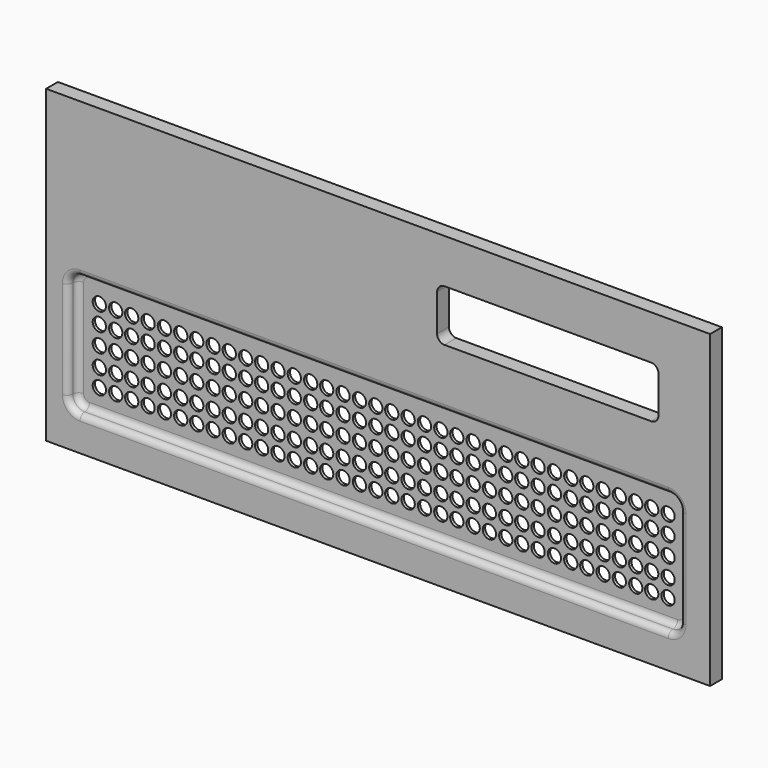
from build123d import *

# Parameters (mm, degrees)
F1_DEPTH = 10
F3_D     = 9
F4_D     = 9
F6_DEPTH = 8
F7_R     = 3.99999


# Not quite as in the source:
# - a fillet or chamfer is up to 0.001 mm smaller than in the source, because OpenCascade refuses the exact size
# - a feature names something its author has since deleted; it is built from what else it names


with BuildPart() as f1:
    # F0 (on Front) → F1 (new body)
    with BuildSketch(Plane.XZ):
        Polygon((0, 210), (0, 0), (450, 0), (450, 210), (265, 210), align=None)
        with BuildLine():
            Line((410, 145), (270, 145))
            ThreePointArc((270, 145), (266.4644660941, 146.4644660941), (265, 150))
            Line((265, 150), (265, 175))
            ThreePointArc((265, 175), (266.4644660941, 178.5355339059), (270, 180))
            Line((270, 180), (410, 180))
            ThreePointArc((410, 180), (413.5355339059, 178.5355339059), (415, 175))
            Line((415, 175), (415, 150))
            ThreePointArc((415, 150), (413.5355339059, 146.4644660941), (410, 145))
        make_face(mode=Mode.SUBTRACT)
    extrude(amount=F1_DEPTH)

    # F3 (through all)
    with Locations(Plane.XZ.offset(10)):
        with Locations((117.7525687963, 75.7827050984), (128.8482453674, 88.015531376), (73.7632680684, 38.015531376), (172.9213949293, 50.0800460577), (51.6047235578, 38.015531376), (150.7628504187, 38.015531376), (150.7628504187, 88.015531376), (128.8482453674, 75.7827050984), (117.7525687963, 38.015531376), (84.8589446396, 38.015531376), (84.8589446396, 63.015531376), (161.8257183582, 38.015531376), (95.6778731197, 75.7827050984), (172.9213949293, 63.015531376), (73.7632680684, 50.0800460577), (172.9213949293, 75.7827050984), (117.7525687963, 88.015531376), (128.8482453674, 38.015531376), (172.9213949293, 38.015531376), (161.8257183582, 63.015531376), (106.7735496908, 50.0800460577), (106.7735496908, 88.015531376), (40.7857950777, 63.015531376), (62.700400129, 63.015531376), (139.6671738476, 88.015531376), (117.7525687963, 50.0800460577), (139.6671738476, 63.015531376), (95.6778731197, 63.015531376), (161.8257183582, 75.7827050984), (106.7735496908, 38.015531376), (73.7632680684, 75.7827050984), (51.6047235578, 63.015531376), (172.9213949293, 88.015531376), (161.8257183582, 88.015531376), (84.8589446396, 75.7827050984), (128.8482453674, 63.015531376), (95.6778731197, 38.015531376), (84.8589446396, 88.015531376), (128.8482453674, 50.0800460577), (51.6047235578, 88.015531376), (62.700400129, 50.0800460577), (62.700400129, 75.7827050984), (51.6047235578, 75.7827050984), (106.7735496908, 63.015531376), (40.7857950777, 75.7827050984), (40.7857950777, 88.015531376), (40.7857950777, 50.0800460577), (29.6901185066, 50.0800460577), (29.6901185066, 63.015531376), (29.6901185066, 75.7827050984), (29.6901185066, 88.015531376), (29.6901185066, 38.015531376), (40.7857950777, 38.015531376), (62.700400129, 88.015531376), (117.7525687963, 63.015531376), (73.7632680684, 88.015531376), (84.8589446396, 50.0800460577), (150.7628504187, 50.0800460577), (51.6047235578, 50.0800460577), (150.7628504187, 75.7827050984), (73.7632680684, 63.015531376), (161.8257183582, 50.0800460577), (95.6778731197, 88.015531376), (150.7628504187, 63.015531376), (62.700400129, 38.015531376), (139.6671738476, 75.7827050984), (139.6671738476, 50.0800460577), (139.6671738476, 38.015531376), (95.6778731197, 50.0800460577), (106.7735496908, 75.7827050984), (183.7403234094, 88.015531376), (194.8359999806, 88.015531376), (205.9469837695, 88.015531376), (217.0426603407, 88.015531376), (227.8615888208, 88.015531376), (238.9572653919, 88.015531376), (194.8359999806, 50.0800460577), (227.8615888208, 63.015531376), (205.9469837695, 63.015531376), (238.9572653919, 75.7827050984), (217.0426603407, 38.015531376), (183.7403234094, 50.0800460577), (238.9572653919, 50.0800460577), (194.8359999806, 38.015531376), (227.8615888208, 75.7827050984), (238.9572653919, 63.015531376), (227.8615888208, 38.015531376), (183.7403234094, 75.7827050984), (194.8359999806, 63.015531376), (205.9469837695, 38.015531376), (194.8359999806, 75.7827050984), (205.9469837695, 75.7827050984), (227.8615888208, 50.0800460577), (205.9469837695, 50.0800460577), (183.7403234094, 63.015531376), (238.9572653919, 38.015531376), (183.7403234094, 38.015531376), (217.0426603407, 75.7827050984), (217.0426603407, 50.0800460577), (217.0426603407, 63.015531376)):
            Hole(F3_D / 2)

    # F4 (through all)
    with Locations(Plane.XZ.offset(10)):
        with Locations((349.1782601923, 88.015531376), (261.1158099025, 63.015531376), (283.0304149538, 63.015531376), (371.0928652436, 88.015531376), (271.9347383827, 38.015531376), (315.9240391105, 88.015531376), (404.0028806776, 38.015531376), (404.0028806776, 63.015531376), (404.0028806776, 50.0800460577), (315.9240391105, 75.7827050984), (338.0825836211, 88.015531376), (349.1782601923, 75.7827050984), (404.0028806776, 88.015531376), (415.0985572487, 63.015531376), (338.0825836211, 63.015531376), (305.1051106304, 50.0800460577), (371.0928652436, 50.0800460577), (359.9971886724, 38.015531376), (415.0985572487, 50.0800460577), (294.0094340593, 88.015531376), (404.0028806776, 75.7827050984), (393.1839521974, 63.015531376), (415.0985572487, 75.7827050984), (327.0197156817, 38.015531376), (294.0094340593, 50.0800460577), (261.1158099025, 88.015531376), (250.0201333314, 50.0800460577), (283.0304149538, 50.0800460577), (382.0882756263, 63.015531376), (338.0825836211, 38.015531376), (349.1782601923, 50.0800460577), (250.0201333314, 75.7827050984), (261.1158099025, 50.0800460577), (359.9971886724, 88.015531376), (305.1051106304, 38.015531376), (382.0882756263, 38.015531376), (327.0197156817, 63.015531376), (271.9347383827, 50.0800460577), (327.0197156817, 75.7827050984), (359.9971886724, 63.015531376), (294.0094340593, 63.015531376), (415.0985572487, 88.015531376), (294.0094340593, 75.7827050984), (315.9240391105, 63.015531376), (382.0882756263, 50.0800460577), (250.0201333314, 63.015531376), (371.0928652436, 75.7827050984), (327.0197156817, 50.0800460577), (338.0825836211, 50.0800460577), (315.9240391105, 38.015531376), (359.9971886724, 75.7827050984), (393.1839521974, 50.0800460577), (315.9240391105, 50.0800460577), (327.0197156817, 88.015531376), (250.0201333314, 88.015531376), (305.1051106304, 75.7827050984), (349.1782601923, 63.015531376), (371.0928652436, 38.015531376), (393.1839521974, 75.7827050984), (283.0304149538, 88.015531376), (371.0928652436, 63.015531376), (283.0304149538, 38.015531376), (305.1051106304, 88.015531376), (305.1051106304, 63.015531376), (261.1158099025, 38.015531376), (283.0304149538, 75.7827050984), (261.1158099025, 75.7827050984), (294.0094340593, 38.015531376), (271.9347383827, 88.015531376), (382.0882756263, 75.7827050984), (349.1782601923, 38.015531376), (271.9347383827, 75.7827050984), (382.0882756263, 88.015531376), (250.0201333314, 38.015531376), (338.0825836211, 75.7827050984), (415.0985572487, 38.015531376), (393.1839521974, 88.015531376), (393.1839521974, 38.015531376), (359.9971886724, 50.0800460577), (271.9347383827, 63.015531376)):
            Hole(F4_D / 2)

    # F5 (on face) → F6 (cut)
    with BuildSketch(Plane.XZ.offset(10)):
        with BuildLine():
            Line((421.6085414886, 105.4098396301), (23.0074847043, 105.4098396301))
            ThreePointArc((23.0074847043, 105.4098396301), (17.3506304548, 103.0666938796), (15.0074847043, 97.4098396301))
            Line((15.0074847043, 97.4098396301), (15.0074847043, 31.1354949325))
            ThreePointArc((15.0074847043, 31.1354949325), (17.3506304548, 25.478640683), (23.0074847043, 23.1354949325))
            Line((23.0074847043, 23.1354949325), (421.6085414886, 23.1354949325))
            ThreePointArc((421.6085414886, 23.1354949325), (427.2653957381, 25.478640683), (429.6085414886, 31.1354949325))
            Line((429.6085414886, 31.1354949325), (429.6085414886, 97.4098396301))
            ThreePointArc((429.6085414886, 97.4098396301), (427.2653957381, 103.0666938796), (421.6085414886, 105.4098396301))
        make_face()
    extrude(amount=-F6_DEPTH, mode=Mode.SUBTRACT)

    # F7 (radius 4 in the source; OpenCascade refuses exactly that, so slightly less here)
    f7_edges = [f1.edges().sort_by_distance(p)[0] for p in [
        (222.308013, -10, 105.40984),
        (17.35063, -10, 103.066694),
        (15.007485, -10, 64.272667),
        (17.35063, -10, 25.478641),
        (222.308013, -10, 23.135495),
        (427.265396, -10, 25.478641),
        (429.608541, -10, 64.272667),
        (427.265396, -10, 103.066694),
        (15.007485, -2, 64.272667),
        (17.35063, -2, 103.066694),
        (222.308013, -2, 105.40984),
    ]]
    fillet(f7_edges, radius=F7_R)


solid = f1.part
